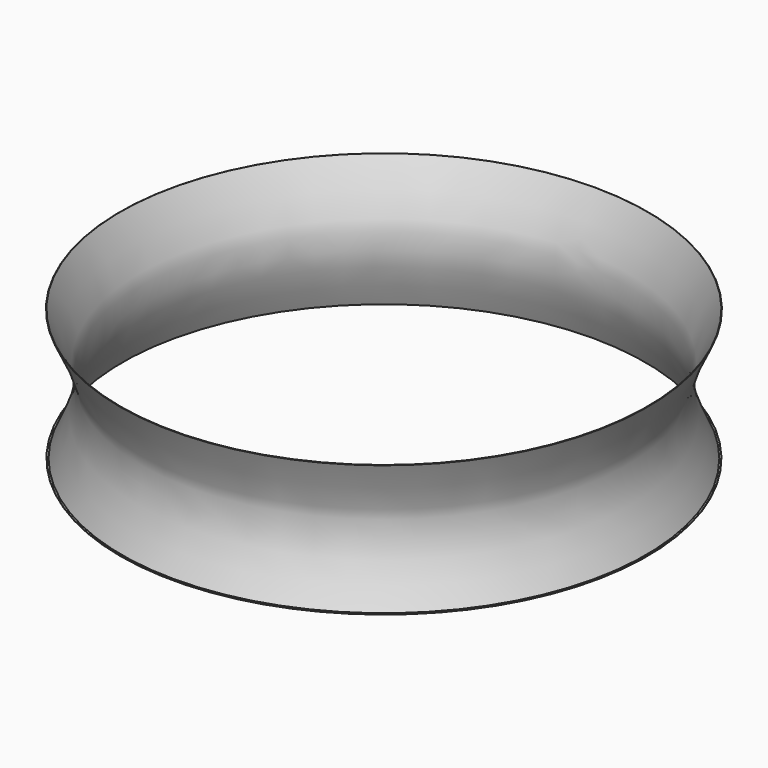
from build123d import *

# Parameters (mm, degrees)
F2_R     = 10
F3_DEPTH = 25


# Not quite as in the source:
# - the dataset's text gives a spline's control points without its knots; the knots are read off the source's solid


with BuildPart() as f1:
    # F0 (on Right) → F1 (revolve)
    with BuildSketch(Plane.YZ):
        with BuildLine():
            Line((5950, 0), (6000, 0))
            Line((6000, 0), (6000, 10))
            Line((6000, 10), (5962.1515274048, 10))
            Line((5962.1515274048, 10), (5959.0849250949, 14.1790113687))
            add(Edge.make_bspline(
                [(6008.9691426502, 2995.5779552105), (5947.599965947, 2871.104114176), (5855.5999367073, 2684.4984216115), (5744.1183321205, 2435.9046667303), (5668.8637968828, 2249.5761908646), (5604.7244604967, 2063.377454738), (5562.8284918667, 1908.3326261904), (5537.611529513, 1784.3742910205), (5523.1892366637, 1691.4440920514), (5515.1957350742, 1614.0336139805), (5511.3861746077, 1552.1217452366), (5509.8627410084, 1505.6972109055), (5509.720751737, 1459.2742365564), (5511.3267686116, 1397.3564694465), (5516.588801064, 1319.928874447), (5527.7696745838, 1226.9614014576), (5548.7087192496, 1102.9323557463), (5585.3337056773, 947.7610861227), (5643.2501808337, 761.356745279), (5712.3644695081, 574.7774830013), (5815.7422120981, 325.8020420574), (5901.726836699, 138.8721243314), (5959.0849250949, 14.1790113687)],
                knots=[0, 0, 0, 0, 0.125, 0.1875, 0.25, 0.3125, 0.375, 0.40625, 0.4375, 0.46875, 0.484375, 0.5, 0.515625, 0.53125, 0.5625, 0.59375, 0.625, 0.6875, 0.75, 0.8125, 0.875, 1, 1, 1, 1], degree=3))
            Line((6008.9691426502, 2995.5779552105), (6000, 3000))
            add(Edge.make_bspline(
                [(6000, 3000), (5753.5582866251, 2500.1473328667), (5262.6048729994, 1504.3566045911), (5721.4695801665, 506.8117008892), (5950, 10)],
                knots=[0, 0, 0, 0, 0.5019655766, 1, 1, 1, 1], degree=3))
            Line((5950, 10), (5950, 0))
        make_face()
    revolve(axis=Axis((0, 0, 1500), (0, 0, 1)))

    # F2 (on face) → F3 (cut)
    with BuildSketch(Plane(origin=(0, 0, 0), x_dir=(1, 0, 0), z_dir=(0, 0, -1))):
        with Locations((-9.2896150255, -5970)):
            Circle(F2_R)
        with Locations((0, 5970)):
            Circle(F2_R)
    extrude(amount=-F3_DEPTH, mode=Mode.SUBTRACT)


solid = f1.part
